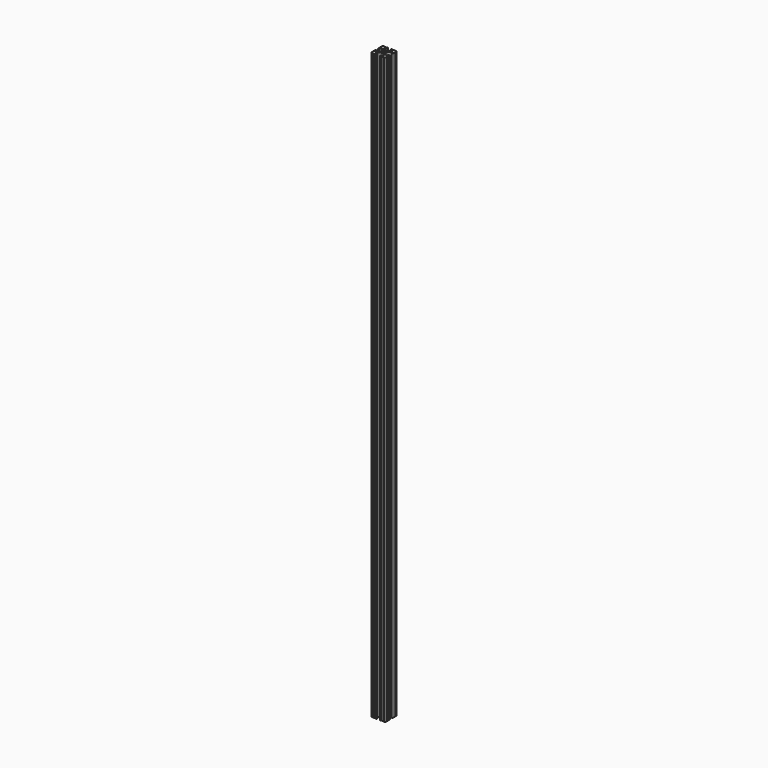
from build123d import *

# Parameters (mm, degrees)
F0_R     = 3.3274
F1_DEPTH = 1524


# Not quite as in the source:
# - ends of sketch curves that miss each other by under 0.0002 mm in the source are joined


with BuildPart() as f1:
    # F0 (on Top) → F1 (new body)
    with BuildSketch(Plane.XY):
        with BuildLine():
            ThreePointArc((-10.0228981846, 12.9147496154), (-10.2183621745, 13.207282149), (-10.287, 13.5523478))
            Line((-10.287, 13.5523478), (-10.287, 14.0843))
            ThreePointArc((-10.287, 14.0843), (-10.0228981846, 14.7218981846), (-9.3853, 14.986))
            Line((-9.3853, 14.986), (-5.6176164, 14.986))
            ThreePointArc((-5.6176164, 14.986), (-4.5190437082, 15.4410437082), (-4.064, 16.5396164))
            Line((-4.064, 16.5396164), (-4.064, 17.4963836))
            ThreePointArc((-4.064, 17.4963836), (-4.5190437082, 18.5949562918), (-5.6176164, 19.05))
            Line((-5.6176164, 19.05), (-7.9741776, 19.05))
            ThreePointArc((-7.9741776, 19.05), (-8.7361776, 18.288), (-9.4981776, 19.05))
            Line((-9.4981776, 19.05), (-14.3277082, 19.05))
            ThreePointArc((-14.3277082, 19.05), (-15.0876, 18.2312564), (-15.8474843511, 19.0499994438))
            ThreePointArc((-15.8474843511, 19.0499994438), (-18.1201820503, 18.1202000102), (-19.0500069498, 15.8475171396))
            ThreePointArc((-19.0500069498, 15.8475171396), (-18.2312564, 15.0876254), (-19.0499994438, 14.3277410489))
            Line((-19.0499994438, 14.3277410489), (-19.05, 9.4960948))
            ThreePointArc((-19.05, 9.4960948), (-18.2312564, 8.736203), (-19.0499994438, 7.9763186489))
            Line((-19.0499994438, 7.9763186489), (-19.05, 5.6176164))
            ThreePointArc((-19.05, 5.6176164), (-18.5949562918, 4.5190437082), (-17.4963836, 4.064))
            Line((-17.4963836, 4.064), (-16.5396164, 4.064))
            ThreePointArc((-16.5396164, 4.064), (-15.4410437082, 4.5190437082), (-14.986, 5.6176164))
            Line((-14.986, 5.6176164), (-14.986, 9.3853508))
            ThreePointArc((-14.986, 9.3853508), (-14.7218981846, 10.0229489846), (-14.0843, 10.2870508))
            Line((-14.0843, 10.2870508), (-13.5160512, 10.2870508))
            ThreePointArc((-13.5160512, 10.2870508), (-13.1709772524, 10.2184095379), (-12.8784403156, 10.0229362846))
            Line((-12.8784403156, 10.0229362846), (-8.1475834, 5.2920646))
            ThreePointArc((-8.1475834, 5.2920646), (-7.1179569965, 3.751117767), (-6.7564, 1.933448))
            Line((-6.7564, 1.933448), (-6.7564, -1.933448))
            ThreePointArc((-6.7564, -1.933448), (-7.1179569965, -3.751117767), (-8.1475842107, -5.2920637893))
            Line((-8.1475842107, -5.2920637893), (-12.878435, -10.0229416))
            ThreePointArc((-12.878435, -10.0229416), (-13.1709772524, -10.2184095379), (-13.5160512, -10.2870508))
            Line((-13.5160512, -10.2870508), (-14.0843, -10.2870508))
            ThreePointArc((-14.0843, -10.2870508), (-14.7218981846, -10.0229489846), (-14.986, -9.3853508))
            Line((-14.986, -9.3853508), (-14.986, -5.6176164))
            ThreePointArc((-14.986, -5.6176164), (-15.4410437082, -4.5190437082), (-16.5396164, -4.064))
            Line((-16.5396164, -4.064), (-17.4963836, -4.064))
            ThreePointArc((-17.4963836, -4.064), (-18.5949562918, -4.5190437082), (-19.05, -5.6176164))
            Line((-19.05, -5.6176164), (-19.05, -7.9763112))
            ThreePointArc((-19.05, -7.9763112), (-18.2312564, -8.736203), (-19.0499994438, -9.4960873511))
            Line((-19.0499994438, -9.4960873511), (-19.05, -14.3277336))
            ThreePointArc((-19.05, -14.3277336), (-18.2312564, -15.0876254), (-19.0499994438, -15.8475097511))
            ThreePointArc((-19.0499994438, -15.8475097511), (-18.1201820503, -18.1202000102), (-15.8474917414, -19.0500067288))
            ThreePointArc((-15.8474917414, -19.0500067288), (-15.0876, -18.2312564), (-14.3277156489, -19.0499994438))
            Line((-14.3277156489, -19.0499994438), (-9.4960694, -19.05))
            ThreePointArc((-9.4960694, -19.05), (-8.7361776, -18.2312564), (-7.9762932489, -19.0499994438))
            Line((-7.9762932489, -19.0499994438), (-5.6176164, -19.05))
            ThreePointArc((-5.6176164, -19.05), (-4.5190437082, -18.5949562918), (-4.064, -17.4963836))
            Line((-4.064, -17.4963836), (-4.064, -16.5396164))
            ThreePointArc((-4.064, -16.5396164), (-4.5190437082, -15.4410437082), (-5.6176164, -14.986))
            Line((-5.6176164, -14.986), (-9.3853, -14.986))
            ThreePointArc((-9.3853, -14.986), (-10.0228981846, -14.7218981846), (-10.287, -14.0843))
            Line((-10.287, -14.0843), (-10.287, -13.5523478))
            ThreePointArc((-10.287, -13.5523478), (-10.2183621745, -13.207282149), (-10.0228981846, -12.9147496154))
            Line((-10.0228981846, -12.9147496154), (-5.2521612, -8.144002))
            ThreePointArc((-5.2521612, -8.144002), (-3.7151749705, -7.1170270023), (-1.9021806, -6.7564))
            Line((-1.9021806, -6.7564), (1.9021806, -6.7564))
            ThreePointArc((1.9021806, -6.7564), (3.7151749705, -7.1170270023), (5.2521573829, -8.1440058171))
            Line((5.2521573829, -8.1440058171), (10.0228908, -12.914757))
            ThreePointArc((10.0228908, -12.914757), (10.2183621745, -13.207282149), (10.287, -13.5523478))
            Line((10.287, -13.5523478), (10.287, -14.0843))
            ThreePointArc((10.287, -14.0843), (10.0228981846, -14.7218981846), (9.3853, -14.986))
            Line((9.3853, -14.986), (5.6176164, -14.986))
            ThreePointArc((5.6176164, -14.986), (4.5190437082, -15.4410437082), (4.064, -16.5396164))
            Line((4.064, -16.5396164), (4.064, -17.4963836))
            ThreePointArc((4.064, -17.4963836), (4.5190437082, -18.5949562918), (5.6176164, -19.05))
            Line((5.6176164, -19.05), (7.9762858, -19.05))
            ThreePointArc((7.9762858, -19.05), (8.7361776, -18.2312564), (9.4960619511, -19.0499994438))
            Line((9.4960619511, -19.0499994438), (14.3277082, -19.05))
            ThreePointArc((14.3277082, -19.05), (15.0876, -18.2312564), (15.8474843511, -19.0499994438))
            ThreePointArc((15.8474843511, -19.0499994438), (18.1201820503, -18.1202000102), (19.0500069498, -15.8475171396))
            ThreePointArc((19.0500069498, -15.8475171396), (18.2312564, -15.0876254), (19.0499994438, -14.3277410489))
            Line((19.0499994438, -14.3277410489), (19.05, -9.4960948))
            ThreePointArc((19.05, -9.4960948), (18.2312564, -8.736203), (19.0499994438, -7.9763186489))
            Line((19.0499994438, -7.9763186489), (19.05, -5.6176164))
            ThreePointArc((19.05, -5.6176164), (18.5949562918, -4.5190437082), (17.4963836, -4.064))
            Line((17.4963836, -4.064), (16.5396164, -4.064))
            ThreePointArc((16.5396164, -4.064), (15.4410437082, -4.5190437082), (14.986, -5.6176164))
            Line((14.986, -5.6176164), (14.986, -9.3853508))
            ThreePointArc((14.986, -9.3853508), (14.7218981846, -10.0229489846), (14.0843, -10.2870508))
            Line((14.0843, -10.2870508), (13.5160512, -10.2870508))
            ThreePointArc((13.5160512, -10.2870508), (13.1709772524, -10.2184095379), (12.8784403156, -10.0229362846))
            Line((12.8784403156, -10.0229362846), (8.1475834, -5.2920646))
            ThreePointArc((8.1475834, -5.2920646), (7.1179569965, -3.751117767), (6.7564, -1.933448))
            Line((6.7564, -1.933448), (6.7564, 1.933448))
            ThreePointArc((6.7564, 1.933448), (7.1179569965, 3.751117767), (8.1475842107, 5.2920637893))
            Line((8.1475842107, 5.2920637893), (12.878435, 10.0229416))
            ThreePointArc((12.878435, 10.0229416), (13.1709772524, 10.2184095379), (13.5160512, 10.2870508))
            Line((13.5160512, 10.2870508), (14.0843, 10.2870508))
            ThreePointArc((14.0843, 10.2870508), (14.7218981846, 10.0229489846), (14.986, 9.3853508))
            Line((14.986, 9.3853508), (14.986, 5.6176164))
            ThreePointArc((14.986, 5.6176164), (15.4410437082, 4.5190437082), (16.5396164, 4.064))
            Line((16.5396164, 4.064), (17.4963836, 4.064))
            ThreePointArc((17.4963836, 4.064), (18.5949562918, 4.5190437082), (19.05, 5.6176164))
            Line((19.05, 5.6176164), (19.05, 7.9763112))
            ThreePointArc((19.05, 7.9763112), (18.2312564, 8.736203), (19.0499994438, 9.4960873511))
            Line((19.0499994438, 9.4960873511), (19.05, 14.3277336))
            ThreePointArc((19.05, 14.3277336), (18.2312564, 15.0876254), (19.0499994438, 15.8475097511))
            ThreePointArc((19.0499994438, 15.8475097511), (18.1201820503, 18.1202000102), (15.8474917414, 19.0500067288))
            ThreePointArc((15.8474917414, 19.0500067288), (15.0876, 18.2312564), (14.3277156489, 19.0499994438))
            Line((14.3277156489, 19.0499994438), (9.4981776, 19.05))
            ThreePointArc((9.4981776, 19.05), (8.7361776, 18.288), (7.9741776, 19.05))
            Line((7.9741776, 19.05), (5.6176164, 19.05))
            ThreePointArc((5.6176164, 19.05), (4.5190437082, 18.5949562918), (4.064, 17.4963836))
            Line((4.064, 17.4963836), (4.064, 16.5396164))
            ThreePointArc((4.064, 16.5396164), (4.5190437082, 15.4410437082), (5.6176164, 14.986))
            Line((5.6176164, 14.986), (9.3853, 14.986))
            ThreePointArc((9.3853, 14.986), (10.0228981846, 14.7218981846), (10.287, 14.0843))
            Line((10.287, 14.0843), (10.287, 13.5523478))
            ThreePointArc((10.287, 13.5523478), (10.2183621745, 13.207282149), (10.0228981846, 12.9147496154))
            Line((10.0228981846, 12.9147496154), (5.2521612, 8.144002))
            ThreePointArc((5.2521612, 8.144002), (3.7151749705, 7.1170270023), (1.9021806, 6.7564))
            Line((1.9021806, 6.7564), (-1.9021806, 6.7564))
            ThreePointArc((-1.9021806, 6.7564), (-3.7151749705, 7.1170270023), (-5.2521573829, 8.1440058171))
            Line((-5.2521573829, 8.1440058171), (-10.0228981846, 12.9147496154))
        make_face()
        Circle(F0_R, mode=Mode.SUBTRACT)
    extrude(amount=F1_DEPTH)


solid = f1.part
